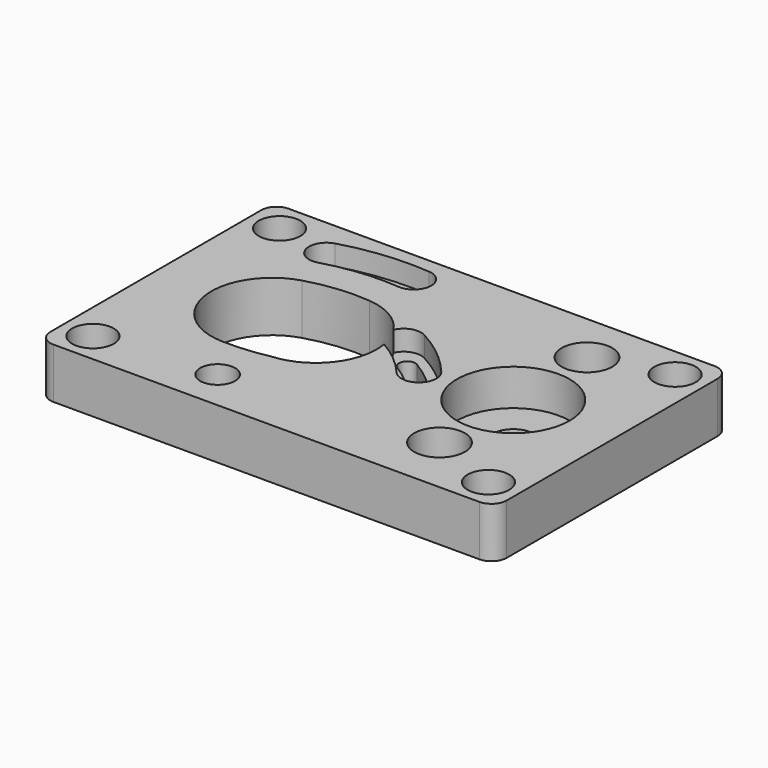
from build123d import *

# Parameters (mm, degrees)
F0_R     = 4.1
F0_R_2   = 3.45
F0_R_3   = 5
F0_R_4   = 11.1
F0_R_5   = 2.1
F0_R_6   = 2.6
F1_DEPTH = 14.96546
F2_DEPTH = 7.2
F3_DEPTH = 10
F4_DEPTH = 6
F5_DEPTH = 5
F6_DEPTH = 4
F8_DEPTH = 5
F9_DEPTH = 4


# Not quite as in the source:
# - a feature of the source that left no trace in its solid (it failed there, or was rolled back) is left out


with BuildPart() as f1:
    # F0 (on Top) → F1 (new body)
    with BuildSketch(Plane.XY):
        with BuildLine():
            Line((40.2978736768, -28.4953018874), (40.2978736768, 23.5046981126))
            ThreePointArc((40.2978736768, 23.5046981126), (39.4191940204, 25.6260184562), (37.2978736768, 26.5046981126))
            Line((37.2978736768, 26.5046981126), (-46.7021263232, 26.5046981126))
            ThreePointArc((-46.7021263232, 26.5046981126), (-48.8234466667, 25.6260184562), (-49.7021263232, 23.5046981126))
            Line((-49.7021263232, 23.5046981126), (-49.7021263232, -28.4953018874))
            ThreePointArc((-49.7021263232, -28.4953018874), (-48.8234466667, -30.616622231), (-46.7021263232, -31.4953018874))
            Line((-46.7021263232, -31.4953018874), (37.2978736768, -31.4953018874))
            ThreePointArc((37.2978736768, -31.4953018874), (39.4191940204, -30.616622231), (40.2978736768, -28.4953018874))
        make_face()
        with Locations((-43.7021263232, -25.4953018874)):
            Circle(F0_R, mode=Mode.SUBTRACT)
        with Locations((-20.7021263232, -23.4953018874)):
            Circle(F0_R_2, mode=Mode.SUBTRACT)
        with Locations((34.2978736768, -25.4953018874)):
            Circle(F0_R, mode=Mode.SUBTRACT)
        with Locations((20.1414857655, -19.8624731614)):
            Circle(F0_R_3, mode=Mode.SUBTRACT)
        with BuildLine():
            ThreePointArc((-27.0610410054, -14.4384550356), (-38.7042248704, -4.0027379443), (-30.1483130342, 9.0840605325))
            ThreePointArc((-30.1483130342, 9.0840605325), (-24.0401350261, 10.2970418321), (-17.812757717, 10.3276042456))
            ThreePointArc((-17.812757717, 10.3276042456), (-12.7496960333, 8.7173903949), (-8.8746668433, 5.0826234101))
            ThreePointArc((-8.8746668433, 5.0826234101), (-6.8344324137, 6.9213428638), (-4.0982992493, 6.6825520261))
            ThreePointArc((-4.0982992493, 6.6825520261), (1.1534268102, 3.1535460469), (5.6424990908, -1.3054605538))
            ThreePointArc((5.6424990908, -1.3054605538), (5.2222958167, -6.1522895109), (0.3747665359, -5.7402438785))
            ThreePointArc((0.3747665359, -5.7402438785), (-3.0402373822, -2.3589951286), (-6.9849022966, 0.3859481464))
            ThreePointArc((-6.9849022966, 0.3859481464), (-9.3764041754, -9.0783459927), (-18.0015595875, -13.6498707823))
            ThreePointArc((-18.0015595875, -13.6498707823), (-22.5078898853, -14.3131084069), (-27.0610410054, -14.4384550356))
        make_face(mode=Mode.SUBTRACT)
        with Locations((-43.7021263232, 20.5046981126)):
            Circle(F0_R, mode=Mode.SUBTRACT)
        with BuildLine():
            ThreePointArc((-33.8725847885, 21.9236712826), (-25.3542994236, 23.5653120636), (-16.6794617957, 23.6232960342))
            ThreePointArc((-16.6794617957, 23.6232960342), (-13.5354362045, 19.8923305986), (-17.2664016401, 16.7483050074))
            ThreePointArc((-17.2664016401, 16.7483050074), (-24.6755091002, 16.698781375), (-31.9509065603, 15.2966694878))
            ThreePointArc((-31.9509065603, 15.2966694878), (-36.2252465717, 17.6493312711), (-33.8725847885, 21.9236712826))
        make_face(mode=Mode.SUBTRACT)
        with Locations((20.1414857655, -1.6874731614)):
            Circle(F0_R_4, mode=Mode.SUBTRACT)
        with Locations((20.1414857655, 16.4875268386)):
            Circle(F0_R_3, mode=Mode.SUBTRACT)
        with Locations((34.2978736768, 20.5046981126)):
            Circle(F0_R, mode=Mode.SUBTRACT)
        with Locations((-43.7021263232, -25.4953018874)):
            Circle(F0_R)
        with Locations((-43.7021263232, -25.4953018874)):
            Circle(F0_R_5, mode=Mode.SUBTRACT)
        with Locations((20.1414857655, -19.8624731614)):
            Circle(F0_R_3)
        with Locations((20.1414857655, -19.8624731614)):
            Circle(F0_R_6, mode=Mode.SUBTRACT)
        with Locations((34.2978736768, -25.4953018874)):
            Circle(F0_R)
        with Locations((34.2978736768, -25.4953018874)):
            Circle(F0_R_5, mode=Mode.SUBTRACT)
        with Locations((34.2978736768, 20.5046981126)):
            Circle(F0_R)
        with Locations((34.2978736768, 20.5046981126)):
            Circle(F0_R_5, mode=Mode.SUBTRACT)
        with Locations((-43.7021263232, 20.5046981126)):
            Circle(F0_R)
        with Locations((-43.7021263232, 20.5046981126)):
            Circle(F0_R_5, mode=Mode.SUBTRACT)
        with BuildLine():
            ThreePointArc((-4.0982992493, 6.6825520261), (-6.8344324137, 6.9213428638), (-8.8746668433, 5.0826234101))
            ThreePointArc((-8.8746668433, 5.0826234101), (-7.6798178788, 2.8348629236), (-6.9849022966, 0.3859481464))
            ThreePointArc((-6.9849022966, 0.3859481464), (-3.0402373822, -2.3589951286), (0.3747665359, -5.7402438785))
            ThreePointArc((0.3747665359, -5.7402438785), (5.2222958167, -6.1522895109), (5.6424990908, -1.3054605538))
            ThreePointArc((5.6424990908, -1.3054605538), (1.1534268102, 3.1535460469), (-4.0982992493, 6.6825520261))
        make_face()
        with BuildLine():
            ThreePointArc((4.228426517, -2.4874076976), (4.0359128199, -4.7419450063), (1.7813755112, -4.5494313092))
            ThreePointArc((1.7813755112, -4.5494313092), (-1.4971898234, -1.2504793297), (-5.2500213098, 1.4969432172))
            Line((-5.2500213098, 1.4969432172), (-5.3461533688, 1.5561161463))
            ThreePointArc((-5.3461533688, 1.5561161463), (-5.8160652882, 3.7640280348), (-3.6190713255, 4.2825930236))
            ThreePointArc((-3.6190713255, 4.2825930236), (-3.6136992043, 4.2793262139), (-3.6083277364, 4.2760583301))
            ThreePointArc((-3.6083277364, 4.2760583301), (0.5902920346, 1.2190394089), (4.228426517, -2.4874076976))
        make_face(mode=Mode.SUBTRACT)
        with Locations((20.1414857655, -1.6874731614)):
            Circle(F0_R_4)
        with Locations((20.1414857655, -1.6874731614)):
            Circle(F0_R, mode=Mode.SUBTRACT)
        with Locations((20.1414857655, 16.4875268386)):
            Circle(F0_R_3)
        with Locations((20.1414857655, 16.4875268386)):
            Circle(F0_R_6, mode=Mode.SUBTRACT)
        with BuildLine():
            ThreePointArc((-17.2664016401, 16.7483050074), (-13.5354362045, 19.8923305986), (-16.6794617957, 23.6232960342))
            ThreePointArc((-16.6794617957, 23.6232960342), (-25.3542994236, 23.5653120636), (-33.8725847885, 21.9236712826))
            ThreePointArc((-33.8725847885, 21.9236712826), (-36.2252465717, 17.6493312711), (-31.9509065603, 15.2966694878))
            ThreePointArc((-31.9509065603, 15.2966694878), (-24.6755091002, 16.698781375), (-17.2664016401, 16.7483050074))
        make_face()
        with BuildLine():
            ThreePointArc((-32.4661391287, 17.0734743169), (-34.4484417427, 18.1645638395), (-33.35735222, 20.1468664535))
            ThreePointArc((-33.35735222, 20.1468664535), (-25.1723049166, 21.7242857196), (-16.836829725, 21.7800013386))
            ThreePointArc((-16.836829725, 21.7800013386), (-15.3787309001, 20.0496985279), (-17.1090337108, 18.591599703))
            ThreePointArc((-17.1090337108, 18.591599703), (-24.8575036072, 18.5398077191), (-32.4661391287, 17.0734743169))
        make_face(mode=Mode.SUBTRACT)
    extrude(amount=-F1_DEPTH)

    # F0 (on Top) → F2 (cut)
    with BuildSketch(Plane.XY):
        with Locations((20.1414857655, -1.6874731614)):
            Circle(F0_R_4)
        with Locations((20.1414857655, -1.6874731614)):
            Circle(F0_R, mode=Mode.SUBTRACT)
    extrude(amount=-F2_DEPTH, mode=Mode.SUBTRACT)

    # F0 (on Top) → F3 (join)
    with BuildSketch(Plane.XY):
        with Locations((-20.7021263232, -23.4953018874)):
            Circle(F0_R_2)
        with BuildLine():
            ThreePointArc((-20.5702775175, -21.9509198451), (-19.5604464975, -22.4469378401), (-19.1521263232, -23.4953018874))
            ThreePointArc((-19.1521263232, -23.4953018874), (-21.6330919297, -24.7345770947), (-21.1338076643, -22.0066275712))
            ThreePointArc((-21.1338076643, -22.0066275712), (-20.9954642962, -21.9733121261), (-20.8546486103, -21.9528243505))
            ThreePointArc((-20.8546486103, -21.9528243505), (-20.7125068335, -21.9453366475), (-20.5702775175, -21.9509198451))
        make_face(mode=Mode.SUBTRACT)
    extrude(amount=-F3_DEPTH)

    # F0 (on Top) → F4 (cut)
    with BuildSketch(Plane.XY):
        with Locations((20.1414857655, 16.4875268386)):
            Circle(F0_R_3)
        with Locations((20.1414857655, 16.4875268386)):
            Circle(F0_R_6, mode=Mode.SUBTRACT)
        with Locations((20.1414857655, -19.8624731614)):
            Circle(F0_R_3)
        with Locations((20.1414857655, -19.8624731614)):
            Circle(F0_R_6, mode=Mode.SUBTRACT)
    extrude(amount=-F4_DEPTH, mode=Mode.SUBTRACT)

    # F0 (on Top) → F5 (cut)
    with BuildSketch(Plane.XY):
        with Locations((-43.7021263232, 20.5046981126)):
            Circle(F0_R)
        with Locations((-43.7021263232, 20.5046981126)):
            Circle(F0_R_5, mode=Mode.SUBTRACT)
        with Locations((-43.7021263232, -25.4953018874)):
            Circle(F0_R)
        with Locations((-43.7021263232, -25.4953018874)):
            Circle(F0_R_5, mode=Mode.SUBTRACT)
        with Locations((34.2978736768, 20.5046981126)):
            Circle(F0_R)
        with Locations((34.2978736768, 20.5046981126)):
            Circle(F0_R_5, mode=Mode.SUBTRACT)
        with Locations((34.2978736768, -25.4953018874)):
            Circle(F0_R)
        with Locations((34.2978736768, -25.4953018874)):
            Circle(F0_R_5, mode=Mode.SUBTRACT)
    extrude(amount=-F5_DEPTH, mode=Mode.SUBTRACT)

    # F0 (on Top) → F6 (cut)
    with BuildSketch(Plane.XY):
        with BuildLine():
            ThreePointArc((-17.2664016401, 16.7483050074), (-13.5354362045, 19.8923305986), (-16.6794617957, 23.6232960342))
            ThreePointArc((-16.6794617957, 23.6232960342), (-25.3542994236, 23.5653120636), (-33.8725847885, 21.9236712826))
            ThreePointArc((-33.8725847885, 21.9236712826), (-36.2252465717, 17.6493312711), (-31.9509065603, 15.2966694878))
            ThreePointArc((-31.9509065603, 15.2966694878), (-24.6755091002, 16.698781375), (-17.2664016401, 16.7483050074))
        make_face()
        with BuildLine():
            ThreePointArc((-32.4661391287, 17.0734743169), (-34.4484417427, 18.1645638395), (-33.35735222, 20.1468664535))
            ThreePointArc((-33.35735222, 20.1468664535), (-25.1723049166, 21.7242857196), (-16.836829725, 21.7800013386))
            ThreePointArc((-16.836829725, 21.7800013386), (-15.3787309001, 20.0496985279), (-17.1090337108, 18.591599703))
            ThreePointArc((-17.1090337108, 18.591599703), (-24.8575036072, 18.5398077191), (-32.4661391287, 17.0734743169))
        make_face(mode=Mode.SUBTRACT)
        with BuildLine():
            ThreePointArc((-4.0982992493, 6.6825520261), (-6.8344324137, 6.9213428638), (-8.8746668433, 5.0826234101))
            ThreePointArc((-8.8746668433, 5.0826234101), (-7.6798178788, 2.8348629236), (-6.9849022966, 0.3859481464))
            ThreePointArc((-6.9849022966, 0.3859481464), (-3.0402373822, -2.3589951286), (0.3747665359, -5.7402438785))
            ThreePointArc((0.3747665359, -5.7402438785), (5.2222958167, -6.1522895109), (5.6424990908, -1.3054605538))
            ThreePointArc((5.6424990908, -1.3054605538), (1.1534268102, 3.1535460469), (-4.0982992493, 6.6825520261))
        make_face()
        with BuildLine():
            ThreePointArc((4.228426517, -2.4874076976), (4.0359128199, -4.7419450063), (1.7813755112, -4.5494313092))
            ThreePointArc((1.7813755112, -4.5494313092), (-1.4971898234, -1.2504793297), (-5.2500213098, 1.4969432172))
            Line((-5.2500213098, 1.4969432172), (-5.3461533688, 1.5561161463))
            ThreePointArc((-5.3461533688, 1.5561161463), (-5.8160652882, 3.7640280348), (-3.6190713255, 4.2825930236))
            ThreePointArc((-3.6190713255, 4.2825930236), (-3.6136992043, 4.2793262139), (-3.6083277364, 4.2760583301))
            ThreePointArc((-3.6083277364, 4.2760583301), (0.5902920346, 1.2190394089), (4.228426517, -2.4874076976))
        make_face(mode=Mode.SUBTRACT)
        with Locations((-20.7021263232, -23.4953018874)):
            Circle(F0_R_2)
        with BuildLine():
            ThreePointArc((-20.5702775175, -21.9509198451), (-19.5604464975, -22.4469378401), (-19.1521263232, -23.4953018874))
            ThreePointArc((-19.1521263232, -23.4953018874), (-21.6330919297, -24.7345770947), (-21.1338076643, -22.0066275712))
            ThreePointArc((-21.1338076643, -22.0066275712), (-20.9954642962, -21.9733121261), (-20.8546486103, -21.9528243505))
            ThreePointArc((-20.8546486103, -21.9528243505), (-20.7125068335, -21.9453366475), (-20.5702775175, -21.9509198451))
        make_face(mode=Mode.SUBTRACT)
    extrude(amount=-F6_DEPTH, mode=Mode.SUBTRACT)

    # F8 (cut): a face of the model
    f8_faces = [f1.faces().sort_by_distance(p)[0] for p in [
        (-2.1196773193, -2.7350856403, -14.96546),
    ]]
    extrude(f8_faces, amount=-F8_DEPTH, mode=Mode.SUBTRACT)

    # F0 (on Top) → F9 (cut)
    with BuildSketch(Plane.XY):
        with Locations((-20.7021263232, -23.4953018874)):
            Circle(F0_R_2)
        with BuildLine():
            ThreePointArc((-20.5702775175, -21.9509198451), (-19.5604464975, -22.4469378401), (-19.1521263232, -23.4953018874))
            ThreePointArc((-19.1521263232, -23.4953018874), (-21.6330919297, -24.7345770947), (-21.1338076643, -22.0066275712))
            ThreePointArc((-21.1338076643, -22.0066275712), (-20.9954642962, -21.9733121261), (-20.8546486103, -21.9528243505))
            ThreePointArc((-20.8546486103, -21.9528243505), (-20.7125068335, -21.9453366475), (-20.5702775175, -21.9509198451))
        make_face(mode=Mode.SUBTRACT)
    extrude(amount=-F9_DEPTH, mode=Mode.SUBTRACT)


solid = f1.part
